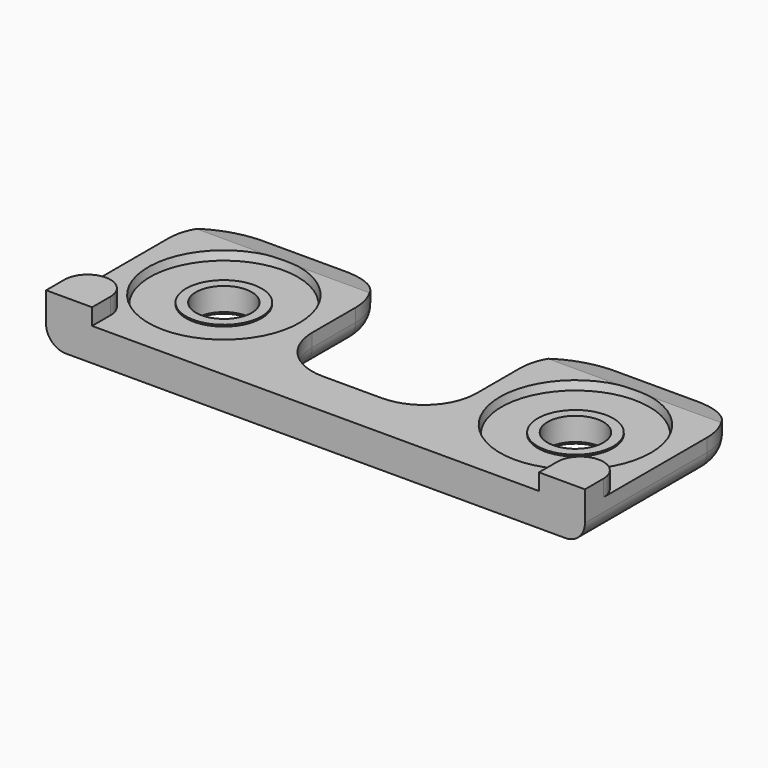
from build123d import *

# Parameters (mm, degrees)
F0_W        = 7
F0_H        = 7
F0_R        = 11.25
F1_DEPTH    = 5
F0_R_2      = 5.75
F0_R_3      = 4.25
F2_DEPTH    = 3.75
F3_DEPTH    = 4
F4_DEPTH    = 7.5
F5_R        = 8
F6_T1_DEPTH = 33.2770199982
F6_T3_DEPTH = 33.2770199982
F7_R        = 3
F8_R        = 3.49999
F9_T2_ANGLE = 270
F9_T4_ANGLE = 270
F9_T6_ANGLE = 90
F9_T8_ANGLE = 90
F10_SIZE    = 0.5


# Not quite as in the source:
# - a fillet or chamfer that OpenCascade refuses, or shapes differently, is made with other operations: its cross-section is extruded or revolved along the edge and cut away or added
# - a fillet or chamfer is up to 0.001 mm smaller than in the source, because OpenCascade refuses the exact size


with BuildPart() as f1:
    # F0 (on Top) → F1 (new body)
    with BuildSketch(Plane.XY):
        with Locations((37.5, 0)):
            Rectangle(F0_W, F0_H)
        Polygon((-34, -3.5), (34, -3.5), (34, 3.5), (41, 3.5), (41, 27.75), (12.5, 27.75), (12.5, 3.5), (-12.5, 3.5), (-12.5, 27.75), (-41, 27.75), (-41, 3.5), (-34, 3.5), align=None)
        with Locations((-26.75, 12.5)):
            Circle(F0_R, mode=Mode.SUBTRACT)
        with Locations((26.75, 12.5)):
            Circle(F0_R, mode=Mode.SUBTRACT)
        with Locations((-37.5, 0)):
            Rectangle(F0_W, F0_H)
    extrude(amount=F1_DEPTH)

    # F0 (on Top) → F2 (join)
    with BuildSketch(Plane.XY):
        with Locations((-26.75, 12.5)):
            Circle(F0_R)
        with Locations((-26.75, 12.5)):
            Circle(F0_R_2, mode=Mode.SUBTRACT)
        with Locations((-26.75, 12.5)):
            Circle(F0_R_2)
        with Locations((-26.75, 12.5)):
            Circle(F0_R_3, mode=Mode.SUBTRACT)
        with Locations((26.75, 12.5)):
            Circle(F0_R)
        with Locations((26.75, 12.5)):
            Circle(F0_R_2, mode=Mode.SUBTRACT)
        with Locations((26.75, 12.5)):
            Circle(F0_R_2)
        with Locations((26.75, 12.5)):
            Circle(F0_R_3, mode=Mode.SUBTRACT)
    extrude(amount=F2_DEPTH)

    # F0 (on Top) → F3 (join)
    with BuildSketch(Plane.XY):
        with Locations((-26.75, 12.5)):
            Circle(F0_R_2)
        with Locations((-26.75, 12.5)):
            Circle(F0_R_3, mode=Mode.SUBTRACT)
        with Locations((26.75, 12.5)):
            Circle(F0_R_2)
        with Locations((26.75, 12.5)):
            Circle(F0_R_3, mode=Mode.SUBTRACT)
    extrude(amount=F3_DEPTH)

    # F0 (on Top) → F4 (join)
    with BuildSketch(Plane.XY):
        with Locations((-37.5, 0)):
            Rectangle(F0_W, F0_H)
        with Locations((37.5, 0)):
            Rectangle(F0_W, F0_H)
    extrude(amount=F4_DEPTH)

    # F5
    f5_edges = [f1.edges().sort_by_distance(p)[0] for p in [
        (-12.5, 3.5, 2.5),
        (12.5, 3.5, 2.5),
        (12.5, 27.75, 2.5),
        (41, 27.75, 2.5),
        (-41, 27.75, 2.5),
        (-12.5, 27.75, 2.5),
    ]]
    fillet(f5_edges, radius=F5_R)

    # F6: chamfer of 1 x 4 on 2 edges, made by hand

    # F6_s2 → F6_t1 (cut)
    with BuildSketch(Plane.YZ.offset(-43.3885099991)):
        Polygon((23.75, 5), (27.75, 4), (27.75, 5), align=None)
    extrude(amount=F6_T1_DEPTH, mode=Mode.SUBTRACT)

    # F6_s4 → F6_t3 (cut)
    with BuildSketch(Plane.YZ.offset(10.1114900009)):
        Polygon((23.75, 5), (27.75, 4), (27.75, 5), align=None)
    extrude(amount=F6_T3_DEPTH, mode=Mode.SUBTRACT)

    # F7
    f7_edges = [f1.edges().sort_by_distance(p)[0] for p in [
        (-26.75, 27.75, 0),
        (41, 8.125, 0),
        (38.656854, 25.406854, 0),
        (26.75, 27.75, 0),
        (-41, 8.125, 0),
        (14.843146, 25.406854, 0),
        (-38.656854, 25.406854, 0),
        (12.5, 15.625, 0),
        (10.156854, 5.843146, 0),
        (-14.843146, 25.406854, 0),
        (0, 3.5, 0),
        (-12.5, 15.625, 0),
        (-10.156854, 5.843146, 0),
    ]]
    fillet(f7_edges, radius=F7_R)

    # F8 (radius 3.5 in the source; OpenCascade refuses exactly that, so slightly less here)
    f8_edges = [f1.edges().sort_by_distance(p)[0] for p in [
        (-34, 3.5, 6.25),
        (-41, 3.5, 6.25),
        (34, 3.5, 6.25),
        (41, 3.5, 6.25),
    ]]
    fillet(f8_edges, radius=F8_R)

    # F9: chamfer of 1.25 x 0.25 on 4 edges, made by hand

    # F9_s1 → F9_t2 (revolve, cut)
    with BuildSketch(Plane.YZ.offset(-26.75)):
        Polygon((24, 5), (23.75, 3.75), (23.75, 5), align=None)
    revolve(axis=Axis((-26.75, 12.5, 5), (0, 0, 1)), revolution_arc=F9_T2_ANGLE, mode=Mode.SUBTRACT)

    # F9_s3 → F9_t4 (revolve, cut)
    with BuildSketch(Plane.YZ.offset(26.75)):
        Polygon((24, 5), (23.75, 3.75), (23.75, 5), align=None)
    revolve(axis=Axis((26.75, 12.5, 5), (0, 0, 1)), revolution_arc=F9_T4_ANGLE, mode=Mode.SUBTRACT)

    # F9_s5 → F9_t6 (revolve, cut)
    with BuildSketch(Plane.XZ.offset(-12.5)):
        Polygon((-15.25, 5), (-15.5, 3.75), (-15.5, 5), align=None)
    revolve(axis=Axis((-26.75, 12.5, 5), (0, 0, 1)), revolution_arc=F9_T6_ANGLE, mode=Mode.SUBTRACT)

    # F9_s7 → F9_t8 (revolve, cut)
    with BuildSketch(Plane.XZ.offset(-12.5)):
        Polygon((38.25, 5), (38, 3.75), (38, 5), align=None)
    revolve(axis=Axis((26.75, 12.5, 5), (0, 0, 1)), revolution_arc=F9_T8_ANGLE, mode=Mode.SUBTRACT)

    # F10
    f10_edges = [f1.edges().sort_by_distance(p)[0] for p in [
        (22.5, 12.5, 0),
        (-31, 12.5, 0),
    ]]
    chamfer(f10_edges, length=F10_SIZE)


solid = f1.part
